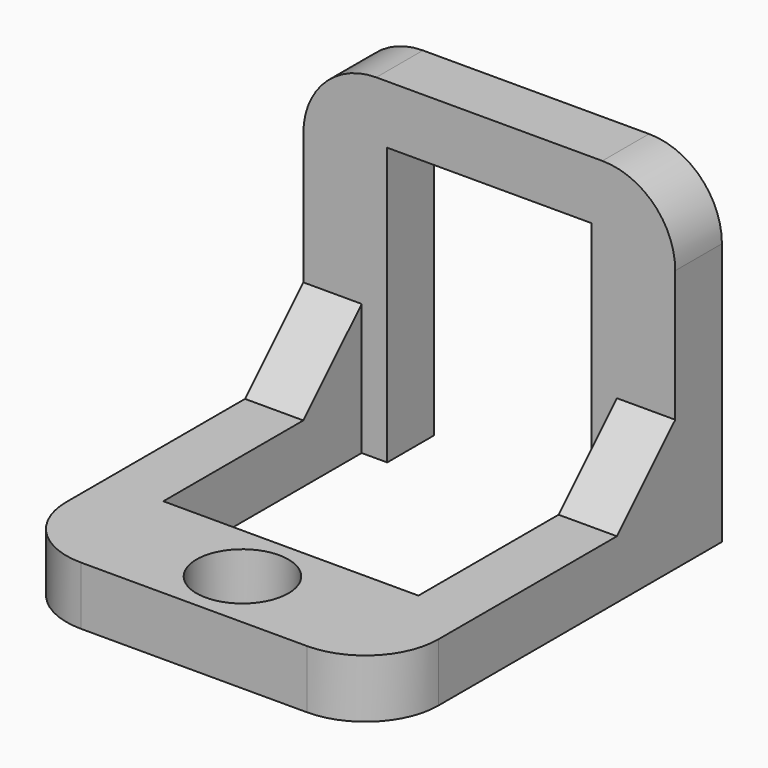
from build123d import *

# Parameters (mm, degrees)
F1_R     = 3.15
F2_DEPTH = 4
F3_DEPTH = 23
F4_DEPTH = 19
F5_R     = 5
F6_SIZE  = 5


# Not quite as in the source:
# - a feature names something its author has since deleted; it is built from what else it names


with BuildPart() as f2:
    # F1 (on Top) → F2 (new body)
    with BuildSketch(Plane.XY):
        Polygon((-4.4541987248, 17.7165100388), (-10.2041987248, 17.7165100388), (-10.2041987248, 13.7165100388), (-6.2041987248, 13.7165100388), (-4.4541987248, 13.7165100388), align=None)
        Polygon((-6.2041987248, 13.7165100388), (-10.2041987248, 13.7165100388), (-10.2041987248, -11.5894424588), (15.2958012752, -11.5894424588), (15.2958012752, 13.7165100388), (11.2958012752, 13.7165100388), (11.2958012752, -3.2953930364), (-6.2041987248, -3.2834899612), align=None)
        with Locations((2.5458012752, -7.4394424588)):
            Circle(F1_R, mode=Mode.SUBTRACT)
        Polygon((9.5458012752, 17.7165100388), (-4.4541987248, 17.7165100388), (-4.4541987248, 13.7165100388), (-3.9542341456, 13.7165100388), (9.5458012752, 13.7165100388), align=None)
        Polygon((15.2958012752, 17.7165100388), (9.5458012752, 17.7165100388), (9.5458012752, 13.7165100388), (11.2958012752, 13.7165100388), (15.2958012752, 13.7165100388), align=None)
    extrude(amount=F2_DEPTH)

    # F1 (on Top) → F3 (join)
    with BuildSketch(Plane.XY):
        Polygon((-4.4541987248, 17.7165100388), (-10.2041987248, 17.7165100388), (-10.2041987248, 13.7165100388), (-6.2041987248, 13.7165100388), (-4.4541987248, 13.7165100388), align=None)
        Polygon((9.5458012752, 17.7165100388), (-4.4541987248, 17.7165100388), (-4.4541987248, 13.7165100388), (-3.9542341456, 13.7165100388), (9.5458012752, 13.7165100388), align=None)
        Polygon((15.2958012752, 17.7165100388), (9.5458012752, 17.7165100388), (9.5458012752, 13.7165100388), (11.2958012752, 13.7165100388), (15.2958012752, 13.7165100388), align=None)
    extrude(amount=F3_DEPTH)

    # F1 (on Top) → F4 (cut)
    with BuildSketch(Plane.XY):
        Polygon((9.5458012752, 17.7165100388), (-4.4541987248, 17.7165100388), (-4.4541987248, 13.7165100388), (-3.9542341456, 13.7165100388), (9.5458012752, 13.7165100388), align=None)
    extrude(amount=F4_DEPTH, mode=Mode.SUBTRACT)

    # F5
    f5_edges = [f2.edges().sort_by_distance(p)[0] for p in [
        (-10.204199, -11.589442, 2),
        (15.295801, -11.589442, 2),
        (15.295801, 15.71651, 23),
        (-10.204199, 15.71651, 23),
    ]]
    fillet(f5_edges, radius=F5_R)

    # F6
    f6_edges = [f2.edges().sort_by_distance(p)[0] for p in [
        (-8.204199, 13.71651, 4),
        (13.295801, 13.71651, 4),
    ]]
    chamfer(f6_edges, length=F6_SIZE)


solid = f2.part
